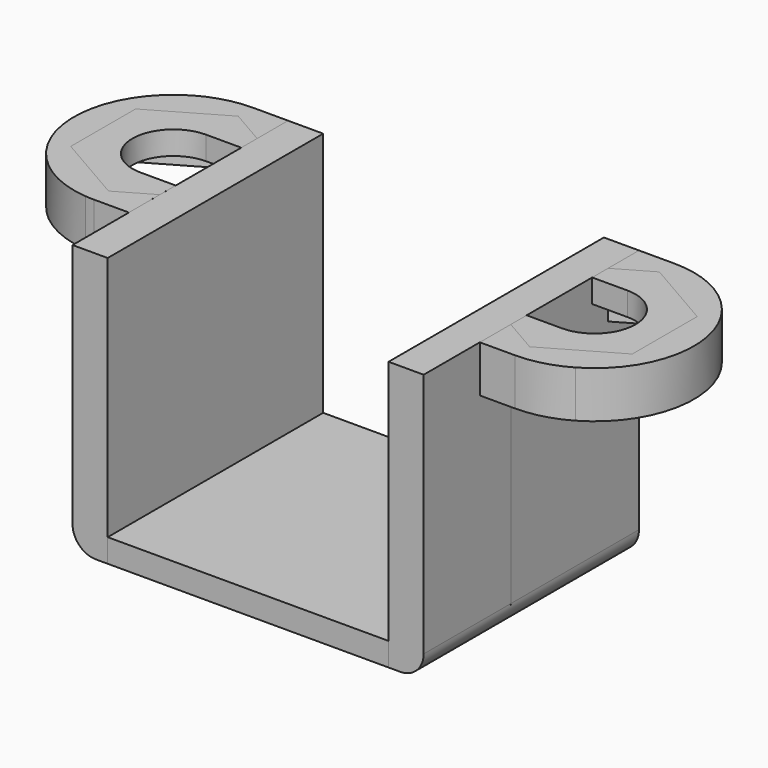
from build123d import *

# Parameters (mm, degrees)
F1_DEPTH = 292.1
F2_DEPTH = 292.1
F3_DEPTH = 50.8
F4_DEPTH = 25.4
F5_DEPTH = 266.7
F6_R     = 25.4
F7_F1_R  = 25.4


with BuildPart() as f1:
    # F0 (on Top) → F1 (new body)
    with BuildSketch(Plane.XY):
        Polygon((-146.9373597216, 152.8665271591), (-146.9381408057, 152.866527607), (-185.0373597216, 152.8883730943), (-185.0373597216, 110.9295088627), (-185.0373597216, 89.3883730943), (-185.0373597216, 0.4883730943), (-185.0373597216, -63.0116269057), (-185.0373597216, -139.4300862217), (-146.9373597216, -139.4300862217), (-146.9373597216, 44.938373096), align=None)
    extrude(amount=-F1_DEPTH)

    # F6
    f6_edges = [f1.edges().sort_by_distance(p)[0] for p in [
        (-185.03736, 6.729143, -292.1),
    ]]
    fillet(f6_edges, radius=F6_R)


with BuildPart() as f1b:
    # F0 (on Top) → F1, piece 2 (new body)
    with BuildSketch(Plane.XY):
        Polygon((195.9625776479, 152.6699137783), (157.8625776479, 152.6699137783), (157.8625776479, 88.7140042905), (157.8625776479, 45.4657096237), (157.8625776479, 0.725823266), (157.8625776479, -139.4300862217), (195.9625776479, -139.4300862217), (195.9625776479, -63.2300862217), (195.9625776479, -21.2796984665), (195.3166993516, -20.89832398), (195.9625776479, -21.2712219881), (195.9625776479, 0.2699137783), (195.9625776479, 89.1699137783), (195.9625776479, 110.7110495466), align=None)
    extrude(amount=-F1_DEPTH)

    # F7: fillet of radius 25.4 on 2 edges, made by hand

    # F7_f1
    f7_f1_edges = [f1b.edges().sort_by_distance(p)[0] for p in [
        (195.9625776479, 65.6993458951, -292.1),
    ]]
    fillet(f7_f1_edges, radius=F7_F1_R)


with BuildPart() as f2:
    # F0 (on Top) → F2 (new body)
    with BuildSketch(Plane.XY):
        Polygon((157.8625776479, 152.6699137783), (5.4626084624, 152.7791434367), (-146.9373597216, 152.8665271591), (-146.9373597216, 44.938373096), (-146.9373597216, -139.4300862217), (157.8625776479, -139.4300862217), (157.8625776479, 0.725823266), (157.8625776479, 45.4657096237), (157.8625776479, 88.7140042905), align=None)
    extrude(amount=-F2_DEPTH)

    # F0 (on Top) → F5 (cut)
    with BuildSketch(Plane.XY):
        Polygon((157.8625776479, 152.6699137783), (5.4626084624, 152.7791434367), (-146.9373597216, 152.8665271591), (-146.9373597216, 44.938373096), (-146.9373597216, -139.4300862217), (157.8625776479, -139.4300862217), (157.8625776479, 0.725823266), (157.8625776479, 45.4657096237), (157.8625776479, 88.7140042905), align=None)
    extrude(amount=-F5_DEPTH, mode=Mode.SUBTRACT)


with BuildPart() as f3:
    # F0 (on Top) → F3 (new body)
    with BuildSketch(Plane.XY):
        with BuildLine():
            Line((-276.9895869982, 101.8443908913), (-276.9895869982, 138.4965908913))
            ThreePointArc((-276.9895869982, 138.4965908913), (-331.0873597064, 44.9401852075), (-276.9927280161, -48.6180366586))
            Line((-276.9927280161, -48.6180366586), (-276.9927280161, -11.954959134))
            Line((-276.9927280161, -11.954959134), (-299.3526036167, 0.9578911619))
            Line((-299.3526036167, 0.9578911619), (-299.3428364707, 88.9455391374))
            Line((-299.3428364707, 88.9455391374), (-276.9895869982, 101.8443908913))
        make_face()
        with BuildLine():
            Line((-185.0373597216, 110.9295088627), (-185.0373597216, 152.8883730943))
            Line((-185.0373597216, 152.8883730943), (-223.1373597216, 152.8883730943))
            ThreePointArc((-223.1373597216, 152.8883730943), (-251.0084279539, 149.2283824701), (-276.9895869982, 138.4965908913))
            Line((-276.9895869982, 138.4965908913), (-276.9895869982, 101.8443908913))
            Line((-276.9895869982, 101.8443908913), (-223.1400223154, 132.9180633213))
            Line((-223.1400223154, 132.9180633213), (-185.0373597216, 110.9295088627))
        make_face()
        with BuildLine():
            Line((-276.9927280161, -11.954959134), (-276.9927280161, -48.6180366586))
            ThreePointArc((-276.9927280161, -48.6180366586), (-255.6304137058, -58.0053199751), (-232.7499348539, -62.5827917958))
            ThreePointArc((-232.7499348539, -62.5827917958), (-227.9484276962, -62.9043648389), (-223.1373597216, -63.0116269057))
            Line((-223.1373597216, -63.0116269057), (-185.0373597216, -63.0116269057))
            Line((-185.0373597216, -63.0116269057), (-185.0583889285, -21.0581061103))
            Line((-185.0583889285, -21.0581061103), (-223.1575768981, -43.0448122021))
            Line((-223.1575768981, -43.0448122021), (-276.9927280161, -11.954959134))
        make_face()
    extrude(amount=-F3_DEPTH)


with BuildPart() as f3b:
    # F0 (on Top) → F3, piece 2 (new body)
    with BuildSketch(Plane.XY):
        with BuildLine():
            ThreePointArc((234.0625776479, -63.2300862217), (261.9872194499, -59.5557635402), (288.0109044248, -48.7829232802))
            Line((288.0109044248, -48.7829232802), (288.0109044248, -12.1207826238))
            Line((288.0109044248, -12.1207826238), (234.0625776496, -43.2682672433))
            Line((234.0625776496, -43.2682672433), (195.9625776479, -21.2712219881))
            Line((195.9625776479, -21.2712219881), (195.9625776479, -21.2796984665))
            Line((195.9625776479, -21.2796984665), (195.9625776479, -63.2300862217))
            Line((195.9625776479, -63.2300862217), (234.0625776479, -63.2300862217))
        make_face()
        with BuildLine():
            ThreePointArc((288.0109044248, -48.7829232802), (342.0125776479, 44.7199137783), (288.0109044248, 138.2227508367))
            Line((288.0109044248, 138.2227508367), (288.0109044248, 101.5614174512))
            Line((288.0109044248, 101.5614174512), (310.2626497377, 88.71453279))
            Line((310.2626497377, 88.71453279), (310.2624181697, 0.7263013092))
            Line((310.2624181697, 0.7263013092), (288.0109044248, -12.1207826238))
            Line((288.0109044248, -12.1207826238), (288.0109044248, -48.7829232802))
        make_face()
        with BuildLine():
            Line((234.0625776479, 152.6699137783), (195.9625776479, 152.6699137783))
            Line((195.9625776479, 152.6699137783), (195.9625776479, 110.7110495466))
            Line((195.9625776479, 110.7110495466), (234.0625776479, 132.7080948028))
            Line((234.0625776479, 132.7080948028), (288.0109044248, 101.5614174512))
            Line((288.0109044248, 101.5614174512), (288.0109044248, 138.2227508367))
            ThreePointArc((288.0109044248, 138.2227508367), (261.9872194499, 148.9955910967), (234.0625776479, 152.6699137783))
        make_face()
    extrude(amount=-F3_DEPTH)


with BuildPart() as f4:
    # F0 (on Top) → F4 (new body)
    with BuildSketch(Plane.XY):
        with BuildLine():
            Line((234.0625776479, 132.7080948028), (195.9625776479, 110.7110495466))
            Line((195.9625776479, 110.7110495466), (195.9625776479, 89.1699137783))
            Line((195.9625776479, 89.1699137783), (234.0625776479, 89.1699137783))
            ThreePointArc((234.0625776479, 89.1699137783), (278.5125776479, 44.7199137783), (234.0625776479, 0.2699137783))
            Line((234.0625776479, 0.2699137783), (195.9625776479, 0.2699137783))
            Line((195.9625776479, 0.2699137783), (195.9625776479, -21.2712219881))
            Line((195.9625776479, -21.2712219881), (234.0625776496, -43.2682672433))
            Line((234.0625776496, -43.2682672433), (288.0109044248, -12.1207826238))
            Line((288.0109044248, -12.1207826238), (310.2624181697, 0.7263013092))
            Line((310.2624181697, 0.7263013092), (310.2626497377, 88.71453279))
            Line((310.2626497377, 88.71453279), (288.0109044248, 101.5614174512))
            Line((288.0109044248, 101.5614174512), (234.0625776479, 132.7080948028))
        make_face()
    extrude(amount=-F4_DEPTH)


with BuildPart() as f4b:
    # F0 (on Top) → F4, piece 2 (new body)
    with BuildSketch(Plane.XY):
        with BuildLine():
            Line((-185.0373597216, 89.3883730943), (-185.0373597216, 110.9295088627))
            Line((-185.0373597216, 110.9295088627), (-223.1400223154, 132.9180633213))
            Line((-223.1400223154, 132.9180633213), (-276.9895869982, 101.8443908913))
            Line((-276.9895869982, 101.8443908913), (-299.3428364707, 88.9455391374))
            Line((-299.3428364707, 88.9455391374), (-299.3526036167, 0.9578911619))
            Line((-299.3526036167, 0.9578911619), (-276.9927280161, -11.954959134))
            Line((-276.9927280161, -11.954959134), (-223.1575768981, -43.0448122021))
            Line((-223.1575768981, -43.0448122021), (-185.0583889285, -21.0581061103))
            Line((-185.0583889285, -21.0581061103), (-185.0373597216, 0.4883730943))
            Line((-185.0373597216, 0.4883730943), (-223.1373597216, 0.4883730943))
            ThreePointArc((-223.1373597216, 0.4883730943), (-267.5873597216, 44.9383730943), (-223.1373597216, 89.3883730943))
            Line((-223.1373597216, 89.3883730943), (-185.0373597216, 89.3883730943))
        make_face()
    extrude(amount=-F4_DEPTH)


solid = Compound([f1.part, f1b.part, f2.part, f3.part, f3b.part, f4.part, f4b.part])
